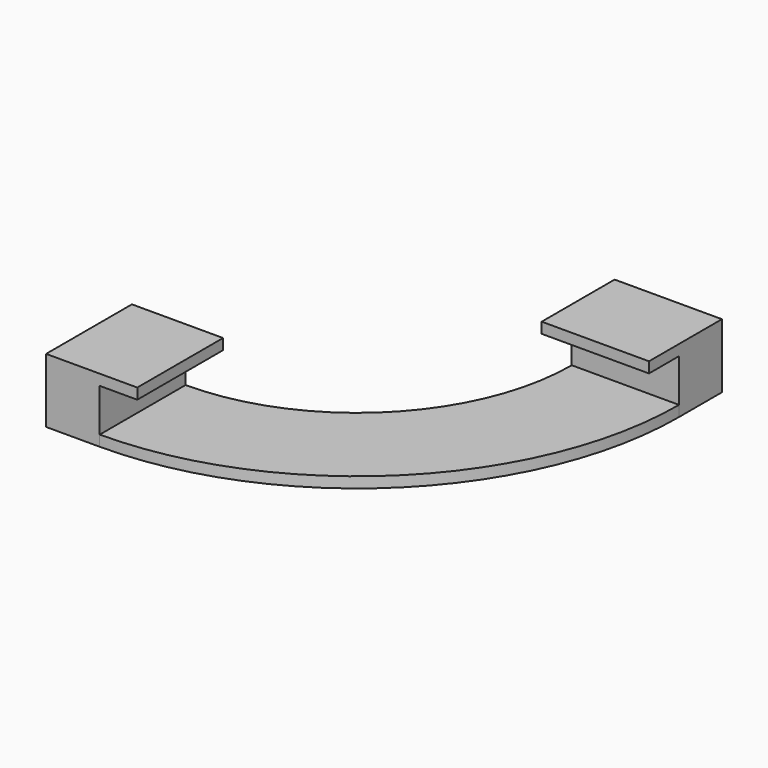
from build123d import *

# Parameters (mm, degrees)
F1_DEPTH = 1
F2_W     = 10
F2_H     = 5
F2_W_2   = 5
F2_H_2   = 10
F3_DEPTH = 5
F5_W     = 10
F5_H     = 1
F6_DEPTH = 3.5
F4_W     = 10
F4_H     = 1
F7_DEPTH = 3.5


with BuildPart() as f1:
    # F0 (on Top) → F1 (new body)
    with BuildSketch(Plane.XY):
        with BuildLine():
            Line((30, 0), (20, 0))
            ThreePointArc((20, 0), (14.1421356237, -14.1421356237), (0, -20))
            Line((0, -20), (0, -25))
            Line((0, -25), (0, -30))
            ThreePointArc((0, -30), (21.2132034356, -21.2132034356), (30, 0))
        make_face()
        with BuildLine():
            Line((20, 5), (20, 0))
            Line((20, 0), (30, 0))
            ThreePointArc((30, 0), (29.8949156836, 2.5087878084), (29.5803989155, 5))
            Line((29.5803989155, 5), (20, 5))
        make_face()
        with BuildLine():
            Line((0, -25), (0, -20))
            Line((0, -20), (-5, -20))
            Line((-5, -20), (-5, -29.5803989155))
            ThreePointArc((-5, -29.5803989155), (-2.5087878084, -29.8949156836), (0, -30))
            Line((0, -30), (0, -25))
        make_face()
        with BuildLine():
            ThreePointArc((29.5803989155, 5), (29.8949156836, 2.5087878084), (30, 0))
            Line((30, 0), (30, 5))
            Line((30, 5), (29.5803989155, 5))
        make_face()
        with BuildLine():
            Line((-5, -30), (0, -30))
            ThreePointArc((0, -30), (-2.5087878084, -29.8949156836), (-5, -29.5803989155))
            Line((-5, -29.5803989155), (-5, -30))
        make_face()
    extrude(amount=F1_DEPTH)

    # F2 (on face) → F3 (join)
    with BuildSketch(Plane.XY.offset(1)):
        with Locations((25, 2.5)):
            Rectangle(F2_W, F2_H)
        with Locations((-2.5, -25)):
            Rectangle(F2_W_2, F2_H_2)
    extrude(amount=F3_DEPTH)

    # F5 (on face) → F6 (join)
    with BuildSketch(Plane.YZ):
        with Locations((-25, 5.5)):
            Rectangle(F5_W, F5_H)
    extrude(amount=F6_DEPTH)

    # F4 (on face) → F7 (join)
    with BuildSketch(Plane.XZ):
        with Locations((25, 5.5)):
            Rectangle(F4_W, F4_H)
    extrude(amount=F7_DEPTH)


solid = f1.part
